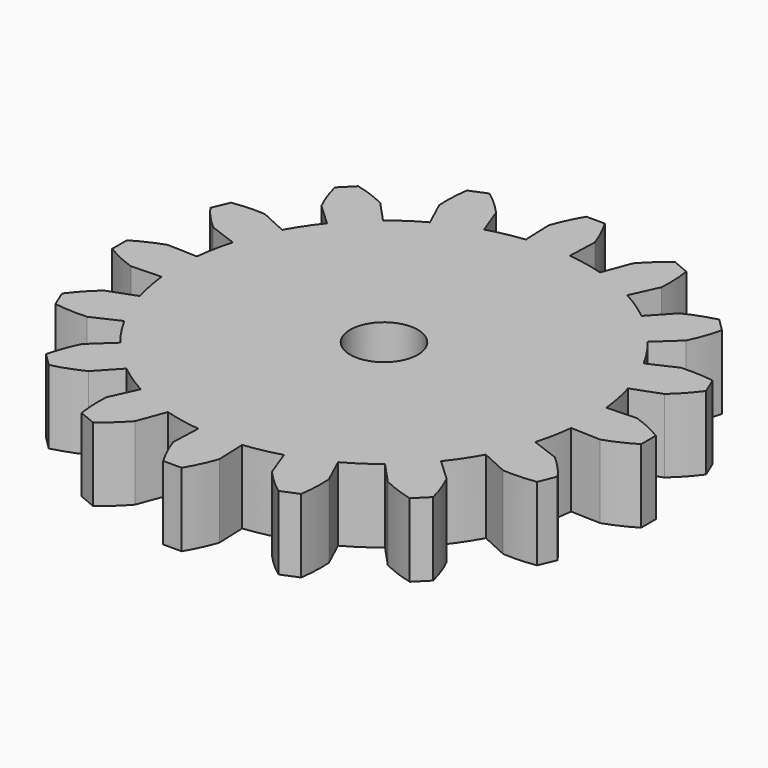
from build123d import *

# Parameters (mm, degrees)
F0_R            = 17.78
F0_R_2          = 2.921
F1_DEPTH        = 6.35
F3_DEPTH        = 6.35
F3_COPIES_COUNT = 16


# Not quite as in the source:
# - a pattern or mirror of a feature is missing from the dataset's text; its kind, count and spacing are read off the source's solid


with BuildPart() as f1:
    # F0 (on Top) → F1 (new body)
    with BuildSketch(Plane.XY):
        Circle(F0_R)
        Circle(F0_R_2, mode=Mode.SUBTRACT)
    extrude(amount=F1_DEPTH)

    # F2 (on face) → F3 (join)
    with BuildSketch(Plane.XY.offset(6.35)):
        with BuildLine():
            Line((1.8639226102, 16.8154710155), (1.9928398674, 20.2606273541))
            ThreePointArc((1.9928398674, 20.2606273541), (1.461833226, 21.5784372569), (0.7936344478, 22.8322719293))
            Line((0.7936344478, 22.8322719293), (-0.0017393364, 22.8322719293))
            Line((-0.0017393364, 22.8322719293), (-0.7971131206, 22.8322719293))
            ThreePointArc((-0.7971131206, 22.8322719293), (-1.4653118988, 21.5784372569), (-1.9963185402, 20.2606273541))
            Line((-1.9963185402, 20.2606273541), (-1.8674012831, 16.8154710155))
            Line((-1.8674012831, 16.8154710155), (-0.0017393364, 16.8154710155))
            Line((-0.0017393364, 16.8154710155), (1.8639226102, 16.8154710155))
        make_face()
    f3 = extrude(amount=-F3_DEPTH)

    # F3_copies: F3 ×16 about axis
    f3_copies_axis = Axis((0, 0, 0), (0, 0, 1))
    for i in range(1, F3_COPIES_COUNT):
        add(f3.rotate(f3_copies_axis, i * 360 / F3_COPIES_COUNT))


solid = f1.part
